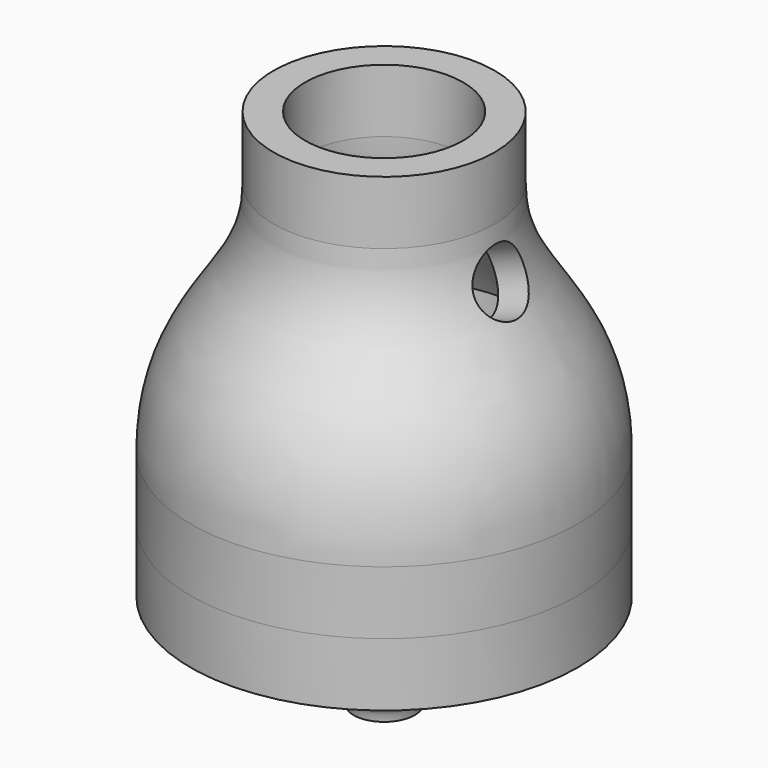
from build123d import *

# Parameters (mm, degrees)
F0_R          = 10.25
F0_R_2        = 8.25
F1_DEPTH      = 1
F0_R_3        = 12.25
F2_DEPTH      = 4
F6_R          = 2
F7_DEPTH      = 2
F7_DEPTH_BACK = 3.8


# Not quite as in the source:
# - ends of sketch curves that miss each other by under 0.0002 mm in the source are joined


with BuildPart() as f1:
    # F0 (on Top) → F1 (new body)
    with BuildSketch(Plane.XY):
        Circle(F0_R)
        Circle(F0_R_2, mode=Mode.SUBTRACT)
    extrude(amount=F1_DEPTH)

    # F0 (on Top) → F2 (join)
    with BuildSketch(Plane.XY):
        Circle(F0_R_3)
        Circle(F0_R, mode=Mode.SUBTRACT)
    extrude(amount=F2_DEPTH)


with BuildPart() as f4:
    # F3 (on Front) → F4 (revolve)
    with BuildSketch(Plane.XZ):
        with BuildLine():
            Line((10.25, 3), (10.25, 4))
            Line((10.25, 4), (10.25, 8))
            add(Edge.make_bspline(
                [(10.25, 8), (10.25, 8.890625), (10.1045119008, 10.43088049), (9.6841800168, 11.8990943349), (9.3594841277, 12.6691561846), (9.2500833857, 12.9054061989)],
                knots=[0, 0, 0, 0, 0.125, 0.25, 0.3076773732, 0.3076773732, 0.3076773732, 0.3076773732], degree=3))
            Line((9.2500833857, 12.9054061989), (9.25, 3))
            Line((9.25, 3), (10.25, 3))
        make_face()
        with BuildLine():
            Line((10.25, 4), (12.25, 4))
            Line((12.25, 4), (12.25, 8))
            add(Edge.make_bspline(
                [(12.25, 8), (12.25, 16), (7, 17), (7, 23)],
                knots=[0, 0, 0, 0, 15.8922150753, 15.8922150753, 15.8922150753, 15.8922150753], degree=3))
            Line((7, 23), (7, 27))
            Line((7, 27), (5, 27))
            Line((5, 27), (5, 23))
            add(Edge.make_bspline(
                [(9.2500833857, 12.9054061989), (9.1223878108, 13.1811637564), (8.7308054078, 13.9421345728), (7.9714226457, 15.1409966434), (6.9629017243, 16.6279097952), (5.967787684, 18.3467518955), (5.1993504319, 20.4411580434), (5, 22.1041666667), (5, 23)],
                knots=[0.3076773732, 0.3076773732, 0.3076773732, 0.3076773732, 0.375, 0.5, 0.625, 0.75, 0.875, 1, 1, 1, 1], degree=3))
            add(Edge.make_bspline(
                [(10.25, 8), (10.25, 8.890625), (10.1045119008, 10.43088049), (9.6841800168, 11.8990943349), (9.3594841277, 12.6691561846), (9.2500833857, 12.9054061989)],
                knots=[0, 0, 0, 0, 0.125, 0.25, 0.3076773732, 0.3076773732, 0.3076773732, 0.3076773732], degree=3))
            Line((10.25, 8), (10.25, 4))
        make_face()
    revolve(axis=Axis((0, 0, 13.5), (0, 0, 1)))

    # F6 (on face) → F7 (cut, two sides)
    with BuildSketch(Plane(origin=(13.0871952127, 0, 4.8021944322), x_dir=(0, -1, 0), z_dir=(-0.9387938378, 0, -0.3444795059))) as f7_sk:
        with Locations((0, 16.1490481287)):
            Circle(F6_R)
    extrude(amount=-F7_DEPTH, mode=Mode.SUBTRACT)
    extrude(f7_sk.sketch, amount=F7_DEPTH_BACK, mode=Mode.SUBTRACT)


with BuildPart() as f9:
    # F8 (on Front) → F9 (revolve)
    with BuildSketch(Plane.XZ):
        with BuildLine():
            add(Edge.make_bspline(
                [(8, 0), (8, -3.3853885252), (1.9431617111, -3.6117282371), (1.9431617111, -6)],
                knots=[0, 0, 0, 0, 8.5255668467, 8.5255668467, 8.5255668467, 8.5255668467], degree=3))
            Line((8, 0), (8, 2))
            Line((8, 2), (0.5, 2))
            Line((0.5, 2), (0.5, -6))
            Line((0.5, -6), (1.9431617111, -6))
        make_face()
    revolve(axis=Axis((0, 0, -2), (0, 0, -1)))


solid = Compound([f1.part, f4.part, f9.part])
